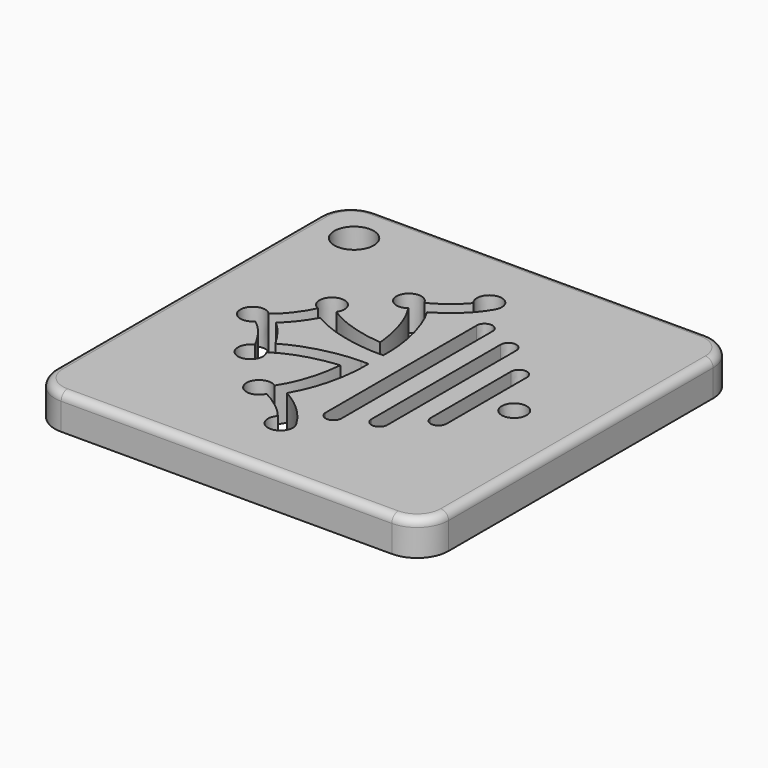
from build123d import *

# Parameters (mm, degrees)
F0_W     = 283.464563
F0_H     = 283.464993
F1_DEPTH = 25
F2_SCALE = 0.088189643
F4_D     = 2.5
F5_R     = 2
F6_R     = 0.5


with BuildPart() as f1:
    # F0 (on Top) → F1 (new body)
    with BuildSketch(Plane.XY):
        with Locations((5e-07, -5e-07)):
            Rectangle(F0_W, F0_H)
        with BuildLine():
            add(Edge.make_bspline(
                [(7.972515, 88.740998), (9.030515, 90.213998), (9.659515, 92.014998), (9.659515, 93.966998)],
                knots=[0, 0, 0, 0, 1, 1, 1, 1], degree=3))
            add(Edge.make_bspline(
                [(-19.344484, 62.948998), (-12.116484, 67.040998), (0.266515, 75.506998), (7.972515, 88.740998)],
                knots=[0, 0, 0, 0, 1, 1, 1, 1], degree=3))
            add(Edge.make_bspline(
                [(-5.780484, 12.037), (-5.772484, 13.232), (-5.745484, 39.625999), (-19.344484, 62.948998)],
                knots=[0, 0, 0, 0, 1, 1, 1, 1], degree=3))
            Line((-5.780484, 12.037), (-5.821484, 6.63))
            Line((-5.821484, 6.63), (-11.225484, 6.581))
            add(Edge.make_bspline(
                [(-62.121483, 20.087999), (-38.811484, 6.5), (-12.425484, 6.563), (-11.225484, 6.581)],
                knots=[0, 0, 0, 0, 1, 1, 1, 1], degree=3))
            add(Edge.make_bspline(
                [(-77.823483, -0.037), (-70.525483, 6.223), (-65.161483, 14.591), (-62.121483, 20.087999)],
                knots=[0, 0, 0, 0, 1, 1, 1, 1], degree=3))
            add(Edge.make_bspline(
                [(-62.119483, -20.183), (-65.159483, -14.681), (-70.524483, -6.302), (-77.823483, -0.037)],
                knots=[0, 0, 0, 0, 1, 1, 1, 1], degree=3))
            add(Edge.make_bspline(
                [(-11.225484, -6.678), (-12.422484, -6.665), (-38.807484, -6.596), (-62.119483, -20.183)],
                knots=[0, 0, 0, 0, 1, 1, 1, 1], degree=3))
            Line((-11.225484, -6.678), (-5.821484, -6.728))
            Line((-5.821484, -6.728), (-5.780484, -12.134))
            add(Edge.make_bspline(
                [(-19.344484, -63.046999), (-5.744484, -39.722999), (-5.772484, -13.329), (-5.780484, -12.134)],
                knots=[0, 0, 0, 0, 1, 1, 1, 1], degree=3))
            add(Edge.make_bspline(
                [(7.972515, -88.837998), (0.265515, -75.603998), (-12.116484, -67.137998), (-19.344484, -63.046999)],
                knots=[0, 0, 0, 0, 1, 1, 1, 1], degree=3))
            add(Edge.make_bspline(
                [(9.659515, -94.063998), (9.659515, -92.111998), (9.030515, -90.310998), (7.972515, -88.837998)],
                knots=[0, 0, 0, 0, 1, 1, 1, 1], degree=3))
            add(Edge.make_bspline(
                [(0.687515, -103.040998), (5.642515, -103.040998), (9.659515, -99.021998), (9.659515, -94.063998)],
                knots=[0, 0, 0, 0, 1, 1, 1, 1], degree=3))
            add(Edge.make_bspline(
                [(-8.284484, -94.063998), (-8.284484, -99.021998), (-4.267484, -103.040998), (0.687515, -103.040998)],
                knots=[0, 0, 0, 0, 1, 1, 1, 1], degree=3))
            add(Edge.make_bspline(
                [(-5.945484, -88.034998), (-7.394484, -89.629998), (-8.284484, -91.739998), (-8.284484, -94.063998)],
                knots=[0, 0, 0, 0, 1, 1, 1, 1], degree=3))
            add(Edge.make_bspline(
                [(-27.730484, -71.031998), (-23.814484, -72.989998), (-13.687484, -78.638998), (-5.945484, -88.034998)],
                knots=[0, 0, 0, 0, 1, 1, 1, 1], degree=3))
            add(Edge.make_bspline(
                [(-35.977484, -76.473998), (-32.277484, -76.473998), (-29.102484, -74.231998), (-27.730484, -71.031998)],
                knots=[0, 0, 0, 0, 1, 1, 1, 1], degree=3))
            add(Edge.make_bspline(
                [(-44.950483, -67.496998), (-44.950483, -72.454998), (-40.933484, -76.473998), (-35.977484, -76.473998)],
                knots=[0, 0, 0, 0, 1, 1, 1, 1], degree=3))
            add(Edge.make_bspline(
                [(-35.977484, -58.520999), (-40.933484, -58.520999), (-44.950483, -62.539999), (-44.950483, -67.496998)],
                knots=[0, 0, 0, 0, 1, 1, 1, 1], degree=3))
            add(Edge.make_bspline(
                [(-30.583484, -60.336999), (-32.086484, -59.201999), (-33.950484, -58.520999), (-35.977484, -58.520999)],
                knots=[0, 0, 0, 0, 1, 1, 1, 1], degree=3))
            add(Edge.make_bspline(
                [(-17.070484, -17.973), (-17.847484, -26.992999), (-20.631484, -45.008999), (-30.583484, -60.336999)],
                knots=[0, 0, 0, 0, 1, 1, 1, 1], degree=3))
            add(Edge.make_bspline(
                [(-59.473483, -31.465999), (-44.193483, -21.53), (-26.110484, -18.75), (-17.070484, -17.973)],
                knots=[0, 0, 0, 0, 1, 1, 1, 1], degree=3))
            add(Edge.make_bspline(
                [(-57.756483, -36.731999), (-57.756483, -34.761999), (-58.398483, -32.946999), (-59.473483, -31.465999)],
                knots=[0, 0, 0, 0, 1, 1, 1, 1], degree=3))
            add(Edge.make_bspline(
                [(-66.728483, -45.707999), (-61.773483, -45.707999), (-57.756483, -41.688999), (-57.756483, -36.731999)],
                knots=[0, 0, 0, 0, 1, 1, 1, 1], degree=3))
            add(Edge.make_bspline(
                [(-75.700483, -36.731999), (-75.700483, -41.688999), (-71.683483, -45.707999), (-66.728483, -45.707999)],
                knots=[0, 0, 0, 0, 1, 1, 1, 1], degree=3))
            add(Edge.make_bspline(
                [(-70.196483, -28.450999), (-73.429483, -29.807999), (-75.700483, -33.003999), (-75.700483, -36.731999)],
                knots=[0, 0, 0, 0, 1, 1, 1, 1], degree=3))
            add(Edge.make_bspline(
                [(-87.852482, -6.169), (-78.876483, -12.254), (-72.437483, -23.955), (-70.196483, -28.450999)],
                knots=[0, 0, 0, 0, 1, 1, 1, 1], degree=3))
            add(Edge.make_bspline(
                [(-94.402482, -9.025), (-91.815482, -9.025), (-89.489482, -7.922), (-87.852482, -6.169)],
                knots=[0, 0, 0, 0, 1, 1, 1, 1], degree=3))
            add(Edge.make_bspline(
                [(-103.375482, -0.049), (-103.375482, -5.006), (-99.358482, -9.025), (-94.402482, -9.025)],
                knots=[0, 0, 0, 0, 1, 1, 1, 1], degree=3))
            add(Edge.make_bspline(
                [(-94.402482, 8.928), (-99.358482, 8.928), (-103.375482, 4.909), (-103.375482, -0.049)],
                knots=[0, 0, 0, 0, 1, 1, 1, 1], degree=3))
            add(Edge.make_bspline(
                [(-87.865482, 6.086), (-89.502482, 7.831), (-91.822482, 8.928), (-94.402482, 8.928)],
                knots=[0, 0, 0, 0, 1, 1, 1, 1], degree=3))
            add(Edge.make_bspline(
                [(-70.197483, 28.354999), (-72.444483, 23.852999), (-78.886483, 12.164), (-87.865482, 6.086)],
                knots=[0, 0, 0, 0, 1, 1, 1, 1], degree=3))
            add(Edge.make_bspline(
                [(-75.700483, 36.634999), (-75.700483, 32.907999), (-73.430483, 29.711999), (-70.197483, 28.354999)],
                knots=[0, 0, 0, 0, 1, 1, 1, 1], degree=3))
            add(Edge.make_bspline(
                [(-66.728483, 45.610999), (-71.683483, 45.610999), (-75.700483, 41.591999), (-75.700483, 36.634999)],
                knots=[0, 0, 0, 0, 1, 1, 1, 1], degree=3))
            add(Edge.make_bspline(
                [(-57.756483, 36.634999), (-57.756483, 41.591999), (-61.773483, 45.610999), (-66.728483, 45.610999)],
                knots=[0, 0, 0, 0, 1, 1, 1, 1], degree=3))
            add(Edge.make_bspline(
                [(-59.473483, 31.368999), (-58.398483, 32.848999), (-57.756483, 34.664999), (-57.756483, 36.634999)],
                knots=[0, 0, 0, 0, 1, 1, 1, 1], degree=3))
            add(Edge.make_bspline(
                [(-17.081484, 17.876999), (-26.126484, 18.654999), (-44.199483, 21.436999), (-59.473483, 31.368999)],
                knots=[0, 0, 0, 0, 1, 1, 1, 1], degree=3))
            add(Edge.make_bspline(
                [(-30.583484, 60.238998), (-20.672484, 44.964999), (-17.870484, 26.912999), (-17.081484, 17.876999)],
                knots=[0, 0, 0, 0, 1, 1, 1, 1], degree=3))
            add(Edge.make_bspline(
                [(-35.977484, 58.423998), (-33.950484, 58.423998), (-32.086484, 59.103998), (-30.583484, 60.238998)],
                knots=[0, 0, 0, 0, 1, 1, 1, 1], degree=3))
            add(Edge.make_bspline(
                [(-44.950483, 67.399998), (-44.950483, 62.442998), (-40.933484, 58.423998), (-35.977484, 58.423998)],
                knots=[0, 0, 0, 0, 1, 1, 1, 1], degree=3))
            add(Edge.make_bspline(
                [(-35.977484, 76.375998), (-40.933484, 76.375998), (-44.950483, 72.357998), (-44.950483, 67.399998)],
                knots=[0, 0, 0, 0, 1, 1, 1, 1], degree=3))
            add(Edge.make_bspline(
                [(-27.733484, 70.939998), (-29.105484, 74.136998), (-32.279484, 76.375998), (-35.977484, 76.375998)],
                knots=[0, 0, 0, 0, 1, 1, 1, 1], degree=3))
            add(Edge.make_bspline(
                [(-5.950484, 87.942998), (-13.675484, 78.590998), (-23.815484, 72.910998), (-27.733484, 70.939998)],
                knots=[0, 0, 0, 0, 1, 1, 1, 1], degree=3))
            add(Edge.make_bspline(
                [(-8.284484, 93.966998), (-8.284484, 91.644998), (-7.396484, 89.536998), (-5.950484, 87.942998)],
                knots=[0, 0, 0, 0, 1, 1, 1, 1], degree=3))
            add(Edge.make_bspline(
                [(0.687515, 102.943997), (-4.267484, 102.943997), (-8.284484, 98.924997), (-8.284484, 93.966998)],
                knots=[0, 0, 0, 0, 1, 1, 1, 1], degree=3))
            add(Edge.make_bspline(
                [(9.659515, 93.966998), (9.659515, 98.924997), (5.642515, 102.943997), (0.687515, 102.943997)],
                knots=[0, 0, 0, 0, 1, 1, 1, 1], degree=3))
        make_face(mode=Mode.SUBTRACT)
        with BuildLine():
            add(Edge.make_bspline(
                [(18.182515, 73.549098), (15.032515, 73.549098), (12.478515, 70.994098), (12.478515, 67.843098)],
                knots=[0, 0, 0, 0, 1, 1, 1, 1], degree=3))
            add(Edge.make_bspline(
                [(23.886515, 67.843098), (23.886515, 70.994098), (21.332515, 73.549098), (18.182515, 73.549098)],
                knots=[0, 0, 0, 0, 1, 1, 1, 1], degree=3))
            Line((23.886515, 67.843098), (23.886515, -68.116898))
            add(Edge.make_bspline(
                [(18.182515, -73.823898), (21.332515, -73.823898), (23.886515, -71.267898), (23.886515, -68.116898)],
                knots=[0, 0, 0, 0, 1, 1, 1, 1], degree=3))
            add(Edge.make_bspline(
                [(12.478515, -68.116898), (12.478515, -71.267898), (15.032515, -73.823898), (18.182515, -73.823898)],
                knots=[0, 0, 0, 0, 1, 1, 1, 1], degree=3))
            Line((12.478515, -68.116898), (12.478515, 67.843098))
        make_face(mode=Mode.SUBTRACT)
        with BuildLine():
            add(Edge.make_bspline(
                [(43.259614, 63.616498), (40.109614, 63.616498), (37.555615, 61.061498), (37.555615, 57.910498)],
                knots=[0, 0, 0, 0, 1, 1, 1, 1], degree=3))
            add(Edge.make_bspline(
                [(48.963614, 57.910498), (48.963614, 61.061498), (46.408614, 63.616498), (43.259614, 63.616498)],
                knots=[0, 0, 0, 0, 1, 1, 1, 1], degree=3))
            Line((48.963614, 57.910498), (48.963614, -58.193499))
            add(Edge.make_bspline(
                [(43.259614, -63.899499), (46.408614, -63.899499), (48.963614, -61.344499), (48.963614, -58.193499)],
                knots=[0, 0, 0, 0, 1, 1, 1, 1], degree=3))
            add(Edge.make_bspline(
                [(37.555615, -58.193499), (37.555615, -61.344499), (40.109614, -63.899499), (43.259614, -63.899499)],
                knots=[0, 0, 0, 0, 1, 1, 1, 1], degree=3))
            Line((37.555615, -58.193499), (37.555615, 57.910498))
        make_face(mode=Mode.SUBTRACT)
        with BuildLine():
            add(Edge.make_bspline(
                [(68.336314, 41.759099), (65.186314, 41.759099), (62.632314, 39.205099), (62.632314, 36.053099)],
                knots=[0, 0, 0, 0, 1, 1, 1, 1], degree=3))
            add(Edge.make_bspline(
                [(74.040314, 36.053099), (74.040314, 39.205099), (71.486314, 41.759099), (68.336314, 41.759099)],
                knots=[0, 0, 0, 0, 1, 1, 1, 1], degree=3))
            Line((74.040314, 36.053099), (74.040314, -36.261899))
            add(Edge.make_bspline(
                [(68.336314, -41.967899), (71.486314, -41.967899), (74.040314, -39.412899), (74.040314, -36.261899)],
                knots=[0, 0, 0, 0, 1, 1, 1, 1], degree=3))
            add(Edge.make_bspline(
                [(62.632314, -36.261899), (62.632314, -39.412899), (65.186314, -41.967899), (68.336314, -41.967899)],
                knots=[0, 0, 0, 0, 1, 1, 1, 1], degree=3))
            Line((62.632314, -36.261899), (62.632314, 36.053099))
        make_face(mode=Mode.SUBTRACT)
        with BuildLine():
            add(Edge.make_bspline(
                [(93.777713, 8.928), (88.822713, 8.928), (84.805713, 4.909), (84.805713, -0.049)],
                knots=[0, 0, 0, 0, 1, 1, 1, 1], degree=3))
            add(Edge.make_bspline(
                [(102.749713, -0.049), (102.749713, 4.909), (98.732713, 8.928), (93.777713, 8.928)],
                knots=[0, 0, 0, 0, 1, 1, 1, 1], degree=3))
            add(Edge.make_bspline(
                [(93.777713, -9.025), (98.732713, -9.025), (102.749713, -5.006), (102.749713, -0.049)],
                knots=[0, 0, 0, 0, 1, 1, 1, 1], degree=3))
            add(Edge.make_bspline(
                [(84.805713, -0.049), (84.805713, -5.006), (88.822713, -9.025), (93.777713, -9.025)],
                knots=[0, 0, 0, 0, 1, 1, 1, 1], degree=3))
        make_face(mode=Mode.SUBTRACT)
    extrude(amount=F1_DEPTH)


with BuildPart() as f1_1:
    # F2: moved
    add(f1.part.scale(F2_SCALE))

    # F4 (through all)
    with Locations(Plane.XY.offset(2.204741075)):
        with Locations((-9.499319263, 9.4993382237)):
            Hole(F4_D / 2)

    # F5
    f5_edges = [f1_1.edges().sort_by_distance(p)[0] for p in [
        (-12.499319, -12.499338, 1.102371),
        (-12.499319, 12.499338, 1.102371),
        (12.499319, -12.499338, 1.102371),
        (12.499319, 12.499338, 1.102371),
    ]]
    fillet(f5_edges, radius=F5_R)

    # F6
    f6_edges = [f1_1.edges().sort_by_distance(p)[0] for p in [
        (-12.499319, 0, 2.204741),
        (-11.913533, 11.913552, 2.204741),
        (-11.913533, -11.913552, 2.204741),
        (0, 12.499338, 2.204741),
        (0, -12.499338, 2.204741),
        (11.913533, 11.913552, 2.204741),
        (11.913533, -11.913552, 2.204741),
        (12.499319, 0, 2.204741),
    ]]
    fillet(f6_edges, radius=F6_R)


solid = f1_1.part
